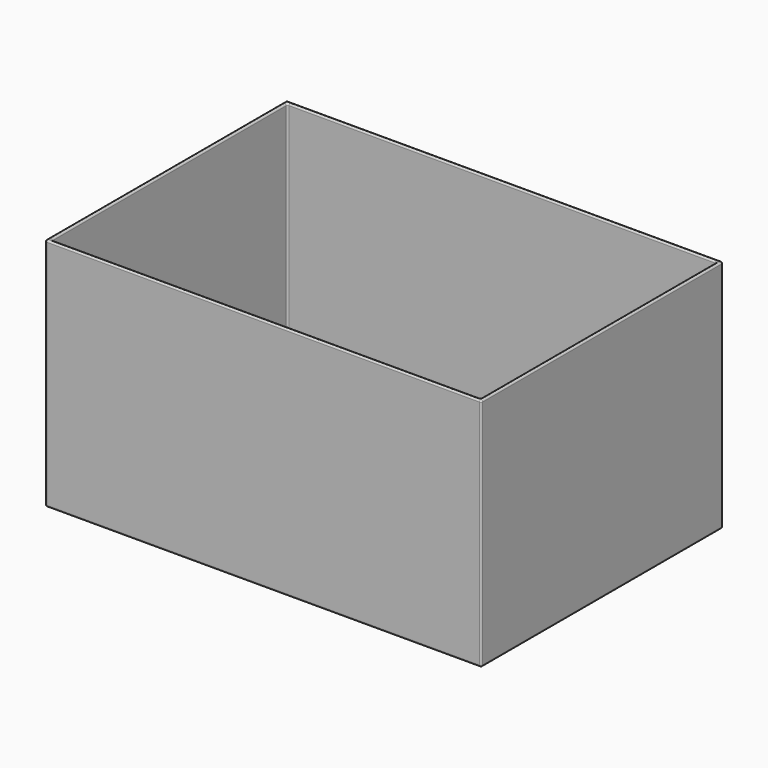
from build123d import *

# Parameters (mm, degrees)
F0_W     = 130
F0_H     = 90
F1_DEPTH = 70
F2_T     = -1
F3_R     = 0.49999


# Not quite as in the source:
# - a fillet or chamfer is up to 0.001 mm smaller than in the source, because OpenCascade refuses the exact size


with BuildPart() as f1:
    # F0 (on Top) → F1 (new body)
    with BuildSketch(Plane.XY):
        Rectangle(F0_W, F0_H)
    extrude(amount=F1_DEPTH)

    # F2
    f2_openings = [f1.faces().sort_by_distance(p)[0] for p in [
        (0, 0, 70),
    ]]
    offset(amount=F2_T, openings=f2_openings)

    # F3 (radius 0.5 in the source; OpenCascade refuses exactly that, so slightly less here)
    f3_edges = [f1.edges().sort_by_distance(p)[0] for p in [
        (-65, -45, 35),
        (65, -45, 35),
        (0, -45, 0),
        (0, -45, 70),
        (-65, 45, 35),
        (-65, 0, 0),
        (-65, 0, 70),
        (65, 45, 35),
        (64, 44, 35.5),
        (-64, 44, 35.5),
        (-64, 0, 70),
        (-64, 0, 1),
        (0, 45, 70),
        (65, 0, 0),
        (65, 0, 70),
        (0, 45, 0),
        (64, -44, 35.5),
        (-64, -44, 35.5),
        (0, -44, 1),
        (0, -44, 70),
        (0, 44, 1),
        (0, 44, 70),
        (64, 0, 1),
        (64, 0, 70),
    ]]
    fillet(f3_edges, radius=F3_R)


solid = f1.part
